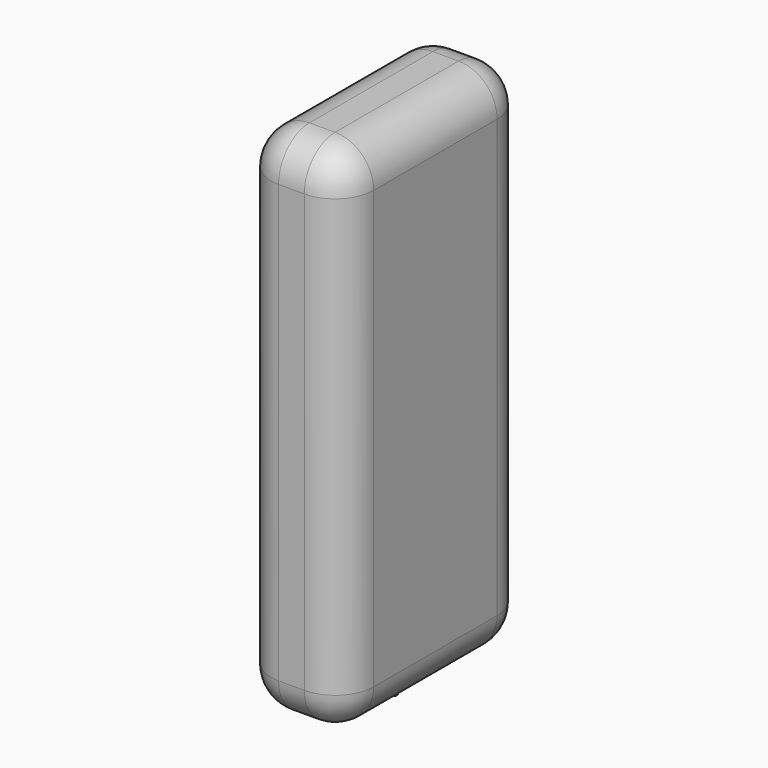
from build123d import *

# Parameters (mm, degrees)
F0_W     = 50.8
F0_H     = 114.3
F1_DEPTH = 254
F2_R     = 1.905
F3_DEPTH = 6.35
F4_F1_R  = 19.05
F4_F2_R  = 19.05
F4_F3_R  = 19.05
F4_F4_R  = 19.05
F4_F5_R  = 19.0499
F4_F6_R  = 19.05


# Not quite as in the source:
# - a fillet or chamfer is up to 0.001 mm smaller than in the source, because OpenCascade refuses the exact size


with BuildPart() as f1:
    # F0 (on Top) → F1 (new body)
    with BuildSketch(Plane.XY):
        Rectangle(F0_W, F0_H)
    extrude(amount=F1_DEPTH)

    # F2 (on face) → F3 (join)
    with BuildSketch(Plane(origin=(0, 0, 0), x_dir=(1, 0, 0), z_dir=(0, 0, -1))):
        with Locations((4.445, 0)):
            Circle(F2_R)
    extrude(amount=F3_DEPTH)

    # F4: fillet of radius 19.05 on 12 edges, made by hand

    # F4_f1
    f4_f1_edges = [f1.edges().sort_by_distance(p)[0] for p in [
        (25.4, -57.15, 127),
    ]]
    fillet(f4_f1_edges, radius=F4_F1_R)

    # F4_f2
    f4_f2_edges = [f1.edges().sort_by_distance(p)[0] for p in [
        (25.4, 57.15, 127),
    ]]
    fillet(f4_f2_edges, radius=F4_F2_R)

    # F4_f3
    f4_f3_edges = [f1.edges().sort_by_distance(p)[0] for p in [
        (-25.4, -57.15, 127),
    ]]
    fillet(f4_f3_edges, radius=F4_F3_R)

    # F4_f4
    f4_f4_edges = [f1.edges().sort_by_distance(p)[0] for p in [
        (-25.4, 57.15, 127),
    ]]
    fillet(f4_f4_edges, radius=F4_F4_R)

    # F4_f5 (radius 19.05 in the source; OpenCascade refuses exactly that, so slightly less here)
    f4_f5_edges = [f1.edges().sort_by_distance(p)[0] for p in [
        (25.4, 0, 0),
    ]]
    fillet(f4_f5_edges, radius=F4_F5_R)

    # F4_f6
    f4_f6_edges = [f1.edges().sort_by_distance(p)[0] for p in [
        (25.4, 0, 254),
    ]]
    fillet(f4_f6_edges, radius=F4_F6_R)


solid = f1.part
